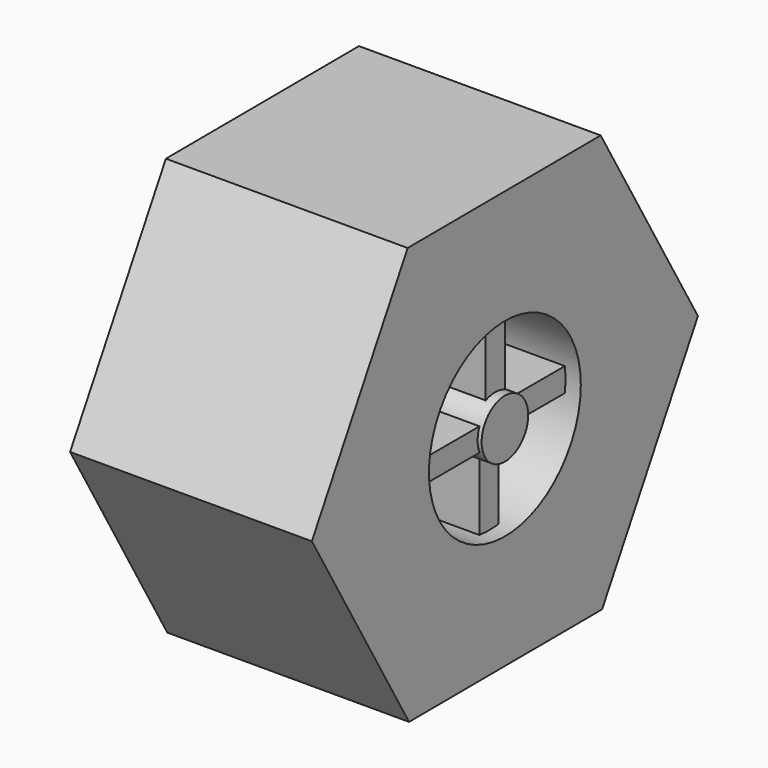
from build123d import *

# Parameters (mm, degrees)
F1_DEPTH  = 76.454
F2_R      = 30.0040123815
F2_R_2    = 9.199471782
F3_DEPTH  = 91.694
F4_W      = 35.7405124232
F4_H      = 7.3380223475
F5_DEPTH  = 75.184
F6_W      = 7.5136311352
F6_H      = 28.0238082632
F7_DEPTH  = 73.406
F8_W      = 7.5136311352
F8_H      = 34.9282254465
F9_DEPTH  = 71.374
F10_W     = 33.3036547527
F10_H     = 7.5136297382
F11_DEPTH = 71.628
F14_R     = 31.6835181621
F15_DEPTH = 5.3


# Not quite as in the source:
# - the program builds the solid bodies; features that only make, move or delete a surface that nothing else refers to are left out


with BuildPart() as f1:
    # F0 (on Right) → F1 (new body)
    with BuildSketch(Plane.YZ):
        Polygon((38.4328120877, -65.9171635344), (76.30234421, 0.3252098396), (37.8695321224, 66.242373374), (-38.4328120877, 65.9171635344), (-76.30234421, -0.3252098396), (-37.8695321224, -66.242373374), align=None)
    extrude(amount=F1_DEPTH)

    # F2 (on Right) → F3 (cut)
    with BuildSketch(Plane.YZ):
        Circle(F2_R)
        Circle(F2_R_2, mode=Mode.SUBTRACT)
    extrude(amount=F3_DEPTH, mode=Mode.SUBTRACT)


with BuildPart() as f5:
    # F4 (on Right) → F5 (new body)
    with BuildSketch(Plane.YZ):
        with Locations((-25.0746384263, 0)):
            Rectangle(F4_W, F4_H)
    extrude(amount=F5_DEPTH)


with BuildPart() as f7:
    # F6 (on Right) → F7 (new body)
    with BuildSketch(Plane.YZ):
        with Locations((0, 19.7994299233)):
            Rectangle(F6_W, F6_H)
    extrude(amount=F7_DEPTH)


with BuildPart() as f9:
    # F8 (on Right) → F9 (new body)
    with BuildSketch(Plane.YZ):
        with Locations((0, -19.7994299233)):
            Rectangle(F8_W, F8_H)
    extrude(amount=F9_DEPTH)


with BuildPart() as f11:
    # F10 (on Right) → F11 (new body)
    with BuildSketch(Plane.YZ):
        with Locations((21.2209261954, 0)):
            Rectangle(F10_W, F10_H)
    extrude(amount=F11_DEPTH)


with BuildPart() as f15:
    # F14 (on Right) → F15 (new body)
    with BuildSketch(Plane.YZ):
        Circle(F14_R)
    extrude(amount=F15_DEPTH)


solid = Compound([f1.part, f5.part, f7.part, f9.part, f11.part, f15.part])
